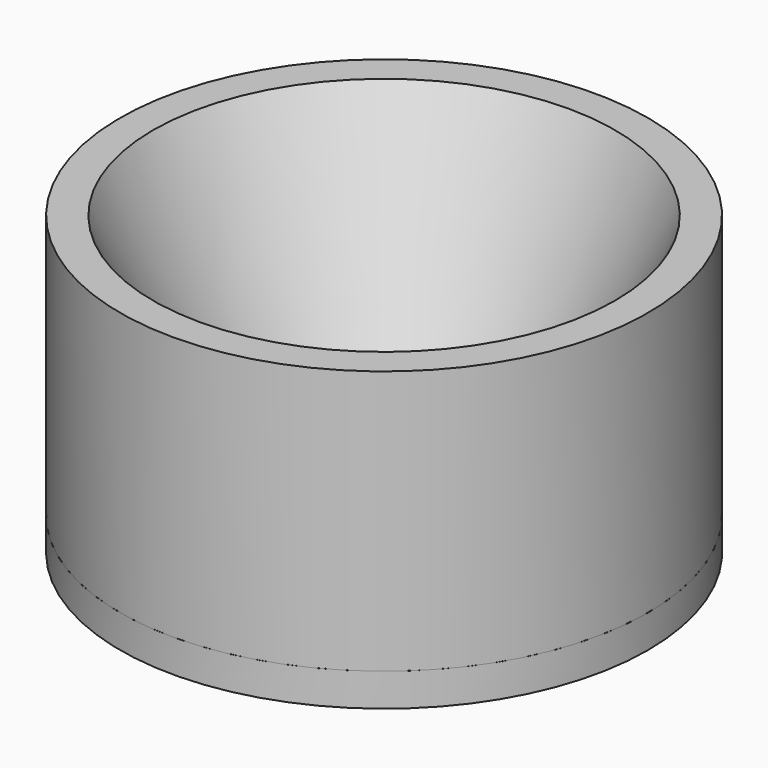
from build123d import *

# Parameters (mm, degrees)
F0_R              = 25.4
F1_DEPTH          = 9.525
F2_R              = 10
F3_DEPTH          = 2
F7_R              = 50.8
F8_DEPTH          = 6.35
F10_D             = 4.4958
F10_DEPTH         = 12.7
F10_CSINK_D       = 9.1186
F10_CSINK_ANGLE   = 82
F10_TIP           = 1.3506745855
F10_2_D           = 4.4958
F10_2_DEPTH       = 12.7
F10_2_CSINK_D     = 9.1186
F10_2_CSINK_ANGLE = 82
F10_2_TIP         = 1.3506745855
F10_3_D           = 4.4958
F10_3_DEPTH       = 12.7
F10_3_CSINK_D     = 9.1186
F10_3_CSINK_ANGLE = 82
F10_3_TIP         = 1.3506745855
F11_D             = 4.0386
F11_DEPTH         = 15.08125
F11_TIP           = 1.213317848
F11_2_D           = 4.0386
F11_2_DEPTH       = 15.08125
F11_2_TIP         = 1.213317848


# Not quite as in the source:
# - a length typed as a fraction of an inch, garbled in the dataset ("3 / 203.2 mm" for 3/8 in), is restored


with BuildPart() as f1:
    # F0 (on Top) → F1 (new body)
    with BuildSketch(Plane.XY):
        Circle(F0_R)
    extrude(amount=F1_DEPTH)

    # F10
    with Locations(Plane(origin=(0, 0, -6.35), x_dir=(1, 0, 0), z_dir=(0, 0, -1))):
        with Locations((0, 38.1), (0, 12.7), (0, -12.7), (0, -38.1)):
            CounterSinkHole(F10_D / 2, F10_CSINK_D / 2, depth=F10_DEPTH, counter_sink_angle=F10_CSINK_ANGLE)
            with Locations((0, 0, -(F10_DEPTH + F10_TIP / 2))):  # 118° drill point
                Cone(0, F10_D / 2, F10_TIP, mode=Mode.SUBTRACT)


with BuildPart() as f3:
    # F2 (on face) → F3 (new body)
    with BuildSketch(Plane.XY.offset(9.525)):
        Circle(F2_R)
    extrude(amount=F3_DEPTH)


with BuildPart() as f6:
    # F5 (on Right) → F6 (revolve)
    with BuildSketch(Plane.YZ):
        Polygon((-50.8, 0), (-25.4, 0), (-25.4, 9.525), (-44.45, 50.8), (-50.8, 50.8), align=None)
    revolve(axis=Axis((0, 0, 35.1485721767), (0, 0, 1)))

    # F10#2
    with Locations(Plane(origin=(0, 0, -6.35), x_dir=(1, 0, 0), z_dir=(0, 0, -1))):
        with Locations((0, 38.1), (0, 12.7), (0, -12.7), (0, -38.1)):
            CounterSinkHole(F10_2_D / 2, F10_2_CSINK_D / 2, depth=F10_2_DEPTH, counter_sink_angle=F10_2_CSINK_ANGLE)
            with Locations((0, 0, -(F10_2_DEPTH + F10_2_TIP / 2))):  # 118° drill point
                Cone(0, F10_2_D / 2, F10_2_TIP, mode=Mode.SUBTRACT)

    # F11
    with Locations(Plane(origin=(0, 0, -6.35), x_dir=(1, 0, 0), z_dir=(0, 0, -1))):
        with Locations((38.1, 0), (-38.1, 0)):
            Hole(F11_D / 2, depth=F11_DEPTH)
            with Locations((0, 0, -(F11_DEPTH + F11_TIP / 2))):  # 118° drill point
                Cone(0, F11_D / 2, F11_TIP, mode=Mode.SUBTRACT)


with BuildPart() as f8:
    # F7 (on face) → F8 (new body)
    with BuildSketch(Plane.XY):
        Circle(F7_R)
    extrude(amount=-F8_DEPTH)

    # F10#3
    with Locations(Plane(origin=(0, 0, -6.35), x_dir=(1, 0, 0), z_dir=(0, 0, -1))):
        with Locations((0, 38.1), (0, 12.7), (0, -12.7), (0, -38.1)):
            CounterSinkHole(F10_3_D / 2, F10_3_CSINK_D / 2, depth=F10_3_DEPTH, counter_sink_angle=F10_3_CSINK_ANGLE)
            with Locations((0, 0, -(F10_3_DEPTH + F10_3_TIP / 2))):  # 118° drill point
                Cone(0, F10_3_D / 2, F10_3_TIP, mode=Mode.SUBTRACT)

    # F11#2
    with Locations(Plane(origin=(0, 0, -6.35), x_dir=(1, 0, 0), z_dir=(0, 0, -1))):
        with Locations((38.1, 0), (-38.1, 0)):
            Hole(F11_2_D / 2, depth=F11_2_DEPTH)
            with Locations((0, 0, -(F11_2_DEPTH + F11_2_TIP / 2))):  # 118° drill point
                Cone(0, F11_2_D / 2, F11_2_TIP, mode=Mode.SUBTRACT)


solid = Compound([f1.part, f3.part, f6.part, f8.part])
